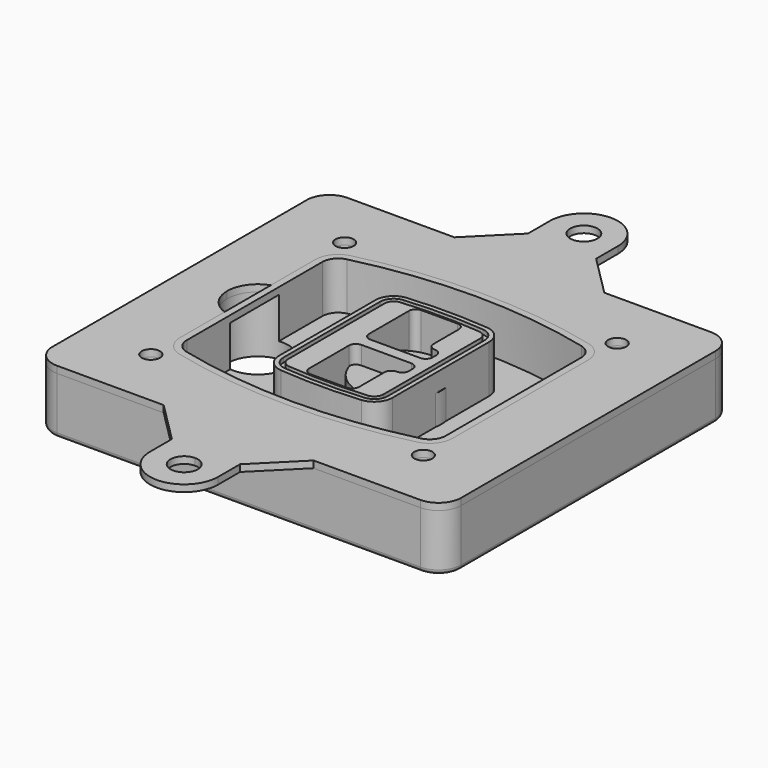
from build123d import *

# Parameters (mm, degrees)
F0_R      = 4
F1_DEPTH  = 25
F2_DEPTH  = 3
F3_DEPTH  = 18
F5_DEPTH  = 21
F6_DEPTH  = 2
F8_DEPTH  = 20
F9_DEPTH  = 16
F10_DEPTH = 25
F7_R      = 6
F7_R_2    = 4
F11_DEPTH = 6
F13_DEPTH = 9
F15_R     = 2
F17_DEPTH = 3
F16_R     = 4
F18_DEPTH = 3


# Not quite as in the source:
# - a feature of the source that left no trace in its solid (it failed there, or was rolled back) is left out
# - a feature names something its author has since deleted; it is built from what else it names


with BuildPart() as f1:
    # F0 (on Top) → F1 (new body)
    with BuildSketch(Plane.XY):
        with BuildLine():
            ThreePointArc((-90, -70), (-87.0710678119, -77.0710678119), (-80, -80))
            Line((-80, -80), (80, -80))
            ThreePointArc((80, -80), (87.0710678119, -77.0710678119), (90, -70))
            Line((90, -70), (90, 70))
            ThreePointArc((90, 70), (87.0710678119, 77.0710678119), (80, 80))
            Line((80, 80), (-80, 80))
            ThreePointArc((-80, 80), (-87.0710678119, 77.0710678119), (-90, 70))
            Line((-90, 70), (-90, -70))
        make_face()
        with Locations((-60, -53.3333333333)):
            Circle(F0_R, mode=Mode.SUBTRACT)
        with Locations((60, -53.3333333333)):
            Circle(F0_R, mode=Mode.SUBTRACT)
        with Locations((-60, 53.3333333333)):
            Circle(F0_R, mode=Mode.SUBTRACT)
        with BuildLine():
            ThreePointArc((-64, 37.2990447398), (-61.0143011354, 45.9411029726), (-53.3306899286, 50.8970778549))
            ThreePointArc((-53.3306899286, 50.8970778549), (0, 57.3333333333), (53.3306899286, 50.8970778549))
            ThreePointArc((53.3306899286, 50.8970778549), (61.0143011354, 45.9411029726), (64, 37.2990447398))
            Line((64, 37.2990447398), (64, -37.2990447398))
            ThreePointArc((64, -37.2990447398), (61.0143011354, -45.9411029726), (53.3306899286, -50.8970778549))
            ThreePointArc((53.3306899286, -50.8970778549), (0, -57.3333333333), (-53.3306899286, -50.8970778549))
            ThreePointArc((-53.3306899286, -50.8970778549), (-61.0143011354, -45.9411029726), (-64, -37.2990447398))
            Line((-64, -37.2990447398), (-64, 37.2990447398))
        make_face(mode=Mode.SUBTRACT)
        with Locations((60, 53.3333333333)):
            Circle(F0_R, mode=Mode.SUBTRACT)
        with BuildLine():
            ThreePointArc((53.3306899286, 50.8970778549), (0, 57.3333333333), (-53.3306899286, 50.8970778549))
            ThreePointArc((-53.3306899286, 50.8970778549), (-61.0143011354, 45.9411029726), (-64, 37.2990447398))
            Line((-64, 37.2990447398), (-64, -37.2990447398))
            ThreePointArc((-64, -37.2990447398), (-61.0143011354, -45.9411029726), (-53.3306899286, -50.8970778549))
            ThreePointArc((-53.3306899286, -50.8970778549), (0, -57.3333333333), (53.3306899286, -50.8970778549))
            ThreePointArc((53.3306899286, -50.8970778549), (61.0143011354, -45.9411029726), (64, -37.2990447398))
            Line((64, -37.2990447398), (64, 37.2990447398))
            ThreePointArc((64, 37.2990447398), (61.0143011354, 45.9411029726), (53.3306899286, 50.8970778549))
        make_face()
        with BuildLine():
            Line((-60, -37.2990447398), (-60, 37.2990447398))
            ThreePointArc((-60, 37.2990447398), (-57.8673579538, 43.4719434775), (-52.3790642347, 47.0119255363))
            ThreePointArc((-52.3790642347, 47.0119255363), (0, 53.3333333333), (52.3790642347, 47.0119255363))
            ThreePointArc((52.3790642347, 47.0119255363), (57.8673579538, 43.4719434775), (60, 37.2990447398))
            Line((60, 37.2990447398), (60, -37.2990447398))
            ThreePointArc((60, -37.2990447398), (57.8673579538, -43.4719434775), (52.3790642347, -47.0119255363))
            ThreePointArc((52.3790642347, -47.0119255363), (0, -53.3333333333), (-52.3790642347, -47.0119255363))
            ThreePointArc((-52.3790642347, -47.0119255363), (-57.8673579538, -43.4719434775), (-60, -37.2990447398))
        make_face(mode=Mode.SUBTRACT)
        with BuildLine():
            ThreePointArc((-52.3790642347, 47.0119255363), (-57.8673579538, 43.4719434775), (-60, 37.2990447398))
            Line((-60, 37.2990447398), (-60, -37.2990447398))
            ThreePointArc((-60, -37.2990447398), (-57.8673579538, -43.4719434775), (-52.3790642347, -47.0119255363))
            ThreePointArc((-52.3790642347, -47.0119255363), (0, -53.3333333333), (52.3790642347, -47.0119255363))
            ThreePointArc((52.3790642347, -47.0119255363), (57.8673579538, -43.4719434775), (60, -37.2990447398))
            Line((60, -37.2990447398), (60, 37.2990447398))
            ThreePointArc((60, 37.2990447398), (57.8673579538, 43.4719434775), (52.3790642347, 47.0119255363))
            ThreePointArc((52.3790642347, 47.0119255363), (0, 53.3333333333), (-52.3790642347, 47.0119255363))
        make_face()
        with BuildLine():
            ThreePointArc((51.6653449643, 44.0980612973), (55.5071505677, 41.6200738562), (57, 37.2990447398))
            Line((57, 37.2990447398), (57, -37.2990447398))
            ThreePointArc((57, -37.2990447398), (55.5071505677, -41.6200738562), (51.6653449643, -44.0980612973))
            ThreePointArc((51.6653449643, -44.0980612973), (0, -50.3333333333), (-51.6653449643, -44.0980612973))
            ThreePointArc((-51.6653449643, -44.0980612973), (-55.5071505677, -41.6200738562), (-57, -37.2990447398))
            Line((-57, -37.2990447398), (-57, 37.2990447398))
            ThreePointArc((-57, 37.2990447398), (-55.5071505677, 41.6200738562), (-51.6653449643, 44.0980612973))
            ThreePointArc((-51.6653449643, 44.0980612973), (0, 50.3333333333), (51.6653449643, 44.0980612973))
        make_face(mode=Mode.SUBTRACT)
        with BuildLine():
            Line((57, -37.2990447398), (57, 37.2990447398))
            ThreePointArc((57, 37.2990447398), (55.5071505677, 41.6200738562), (51.6653449643, 44.0980612973))
            ThreePointArc((51.6653449643, 44.0980612973), (0, 50.3333333333), (-51.6653449643, 44.0980612973))
            ThreePointArc((-51.6653449643, 44.0980612973), (-55.5071505677, 41.6200738562), (-57, 37.2990447398))
            Line((-57, 37.2990447398), (-57, -37.2990447398))
            ThreePointArc((-57, -37.2990447398), (-55.5071505677, -41.6200738562), (-51.6653449643, -44.0980612973))
            ThreePointArc((-51.6653449643, -44.0980612973), (0, -50.3333333333), (51.6653449643, -44.0980612973))
            ThreePointArc((51.6653449643, -44.0980612973), (55.5071505677, -41.6200738562), (57, -37.2990447398))
        make_face()
    extrude(amount=-F1_DEPTH)

    # F0 (on Top) → F2 (join)
    with BuildSketch(Plane.XY):
        with BuildLine():
            ThreePointArc((-52.3790642347, 47.0119255363), (-57.8673579538, 43.4719434775), (-60, 37.2990447398))
            Line((-60, 37.2990447398), (-60, -37.2990447398))
            ThreePointArc((-60, -37.2990447398), (-57.8673579538, -43.4719434775), (-52.3790642347, -47.0119255363))
            ThreePointArc((-52.3790642347, -47.0119255363), (0, -53.3333333333), (52.3790642347, -47.0119255363))
            ThreePointArc((52.3790642347, -47.0119255363), (57.8673579538, -43.4719434775), (60, -37.2990447398))
            Line((60, -37.2990447398), (60, 37.2990447398))
            ThreePointArc((60, 37.2990447398), (57.8673579538, 43.4719434775), (52.3790642347, 47.0119255363))
            ThreePointArc((52.3790642347, 47.0119255363), (0, 53.3333333333), (-52.3790642347, 47.0119255363))
        make_face()
        with BuildLine():
            ThreePointArc((51.6653449643, 44.0980612973), (55.5071505677, 41.6200738562), (57, 37.2990447398))
            Line((57, 37.2990447398), (57, -37.2990447398))
            ThreePointArc((57, -37.2990447398), (55.5071505677, -41.6200738562), (51.6653449643, -44.0980612973))
            ThreePointArc((51.6653449643, -44.0980612973), (0, -50.3333333333), (-51.6653449643, -44.0980612973))
            ThreePointArc((-51.6653449643, -44.0980612973), (-55.5071505677, -41.6200738562), (-57, -37.2990447398))
            Line((-57, -37.2990447398), (-57, 37.2990447398))
            ThreePointArc((-57, 37.2990447398), (-55.5071505677, 41.6200738562), (-51.6653449643, 44.0980612973))
            ThreePointArc((-51.6653449643, 44.0980612973), (0, 50.3333333333), (51.6653449643, 44.0980612973))
        make_face(mode=Mode.SUBTRACT)
    extrude(amount=F2_DEPTH)

    # F0 (on Top) → F3 (cut)
    with BuildSketch(Plane.XY):
        with BuildLine():
            Line((57, -37.2990447398), (57, 37.2990447398))
            ThreePointArc((57, 37.2990447398), (55.5071505677, 41.6200738562), (51.6653449643, 44.0980612973))
            ThreePointArc((51.6653449643, 44.0980612973), (0, 50.3333333333), (-51.6653449643, 44.0980612973))
            ThreePointArc((-51.6653449643, 44.0980612973), (-55.5071505677, 41.6200738562), (-57, 37.2990447398))
            Line((-57, 37.2990447398), (-57, -37.2990447398))
            ThreePointArc((-57, -37.2990447398), (-55.5071505677, -41.6200738562), (-51.6653449643, -44.0980612973))
            ThreePointArc((-51.6653449643, -44.0980612973), (0, -50.3333333333), (51.6653449643, -44.0980612973))
            ThreePointArc((51.6653449643, -44.0980612973), (55.5071505677, -41.6200738562), (57, -37.2990447398))
        make_face()
    extrude(amount=-F3_DEPTH, mode=Mode.SUBTRACT)

    # F4 (on face) → F5 (join, through all)
    with BuildSketch(Plane.XY.offset(3)):
        with BuildLine():
            ThreePointArc((-25, -26.587695628), (-22.8992979869, -31.9912392117), (-17.7004291845, -34.5569740744))
            ThreePointArc((-17.7004291845, -34.5569740744), (0, -35.3333333333), (17.7004291845, -34.5569740744))
            ThreePointArc((17.7004291845, -34.5569740744), (22.8992979869, -31.9912392117), (25, -26.587695628))
            Line((25, -26.587695628), (25, 26.587695628))
            ThreePointArc((25, 26.587695628), (22.8992979869, 31.9912392117), (17.7004291845, 34.5569740744))
            ThreePointArc((17.7004291845, 34.5569740744), (0, 35.3333333333), (-17.7004291845, 34.5569740744))
            ThreePointArc((-17.7004291845, 34.5569740744), (-22.8992979869, 31.9912392117), (-25, 26.587695628))
            Line((-25, 26.587695628), (-25, -26.587695628))
        make_face()
        with BuildLine():
            ThreePointArc((17.5253218884, 32.5646544628), (21.4244734902, 30.6403533158), (23, 26.587695628))
            Line((23, 26.587695628), (23, -26.587695628))
            ThreePointArc((23, -26.587695628), (21.4244734902, -30.6403533158), (17.5253218884, -32.5646544628))
            ThreePointArc((17.5253218884, -32.5646544628), (0, -33.3333333333), (-17.5253218884, -32.5646544628))
            ThreePointArc((-17.5253218884, -32.5646544628), (-21.4244734902, -30.6403533158), (-23, -26.587695628))
            Line((-23, -26.587695628), (-23, 26.587695628))
            ThreePointArc((-23, 26.587695628), (-21.4244734902, 30.6403533158), (-17.5253218884, 32.5646544628))
            ThreePointArc((-17.5253218884, 32.5646544628), (0, 33.3333333333), (17.5253218884, 32.5646544628))
        make_face(mode=Mode.SUBTRACT)
        with BuildLine():
            Line((23, -26.587695628), (23, 26.587695628))
            ThreePointArc((23, 26.587695628), (21.4244734902, 30.6403533158), (17.5253218884, 32.5646544628))
            ThreePointArc((17.5253218884, 32.5646544628), (0, 33.3333333333), (-17.5253218884, 32.5646544628))
            ThreePointArc((-17.5253218884, 32.5646544628), (-21.4244734902, 30.6403533158), (-23, 26.587695628))
            Line((-23, 26.587695628), (-23, -26.587695628))
            ThreePointArc((-23, -26.587695628), (-21.4244734902, -30.6403533158), (-17.5253218884, -32.5646544628))
            ThreePointArc((-17.5253218884, -32.5646544628), (0, -33.3333333333), (17.5253218884, -32.5646544628))
            ThreePointArc((17.5253218884, -32.5646544628), (21.4244734902, -30.6403533158), (23, -26.587695628))
        make_face()
        with BuildLine():
            ThreePointArc((17.3502145923, 30.5723348512), (19.9496489934, 29.2894674198), (21, 26.587695628))
            Line((21, 26.587695628), (21, -26.587695628))
            ThreePointArc((21, -26.587695628), (19.9496489934, -29.2894674198), (17.3502145923, -30.5723348512))
            ThreePointArc((17.3502145923, -30.5723348512), (0, -31.3333333333), (-17.3502145923, -30.5723348512))
            ThreePointArc((-17.3502145923, -30.5723348512), (-19.9496489934, -29.2894674198), (-21, -26.587695628))
            Line((-21, -26.587695628), (-21, 26.587695628))
            ThreePointArc((-21, 26.587695628), (-19.9496489934, 29.2894674198), (-17.3502145923, 30.5723348512))
            ThreePointArc((-17.3502145923, 30.5723348512), (0, 31.3333333333), (17.3502145923, 30.5723348512))
        make_face(mode=Mode.SUBTRACT)
        with BuildLine():
            Line((21, -26.587695628), (21, 26.587695628))
            ThreePointArc((21, 26.587695628), (19.9496489934, 29.2894674198), (17.3502145923, 30.5723348512))
            ThreePointArc((17.3502145923, 30.5723348512), (0, 31.3333333333), (-17.3502145923, 30.5723348512))
            ThreePointArc((-17.3502145923, 30.5723348512), (-19.9496489934, 29.2894674198), (-21, 26.587695628))
            Line((-21, 26.587695628), (-21, -26.587695628))
            ThreePointArc((-21, -26.587695628), (-19.9496489934, -29.2894674198), (-17.3502145923, -30.5723348512))
            ThreePointArc((-17.3502145923, -30.5723348512), (0, -31.3333333333), (17.3502145923, -30.5723348512))
            ThreePointArc((17.3502145923, -30.5723348512), (19.9496489934, -29.2894674198), (21, -26.587695628))
        make_face()
        with BuildLine():
            Line((-8, -2.5), (14, -2.5))
            ThreePointArc((14, -2.5), (16.1213203436, -3.3786796564), (17, -5.5))
            Line((17, -5.5), (17, -7.5))
            ThreePointArc((17, -7.5), (16.1213203436, -9.6213203436), (14, -10.5))
            ThreePointArc((14, -10.5), (11.8786796564, -11.3786796564), (11, -13.5))
            Line((11, -13.5), (11, -27.5))
            ThreePointArc((11, -27.5), (10.1213203436, -29.6213203436), (8, -30.5))
            Line((8, -30.5), (-8, -30.5))
            ThreePointArc((-8, -30.5), (-10.1213203436, -29.6213203436), (-11, -27.5))
            Line((-11, -27.5), (-11, -5.5))
            ThreePointArc((-11, -5.5), (-10.1213203436, -3.3786796564), (-8, -2.5))
        make_face(mode=Mode.SUBTRACT)
        with BuildLine():
            ThreePointArc((-8, 2.5), (-10.1213203436, 3.3786796564), (-11, 5.5))
            Line((-11, 5.5), (-11, 27.5))
            ThreePointArc((-11, 27.5), (-10.1213203436, 29.6213203436), (-8, 30.5))
            Line((-8, 30.5), (8, 30.5))
            ThreePointArc((8, 30.5), (10.1213203436, 29.6213203436), (11, 27.5))
            Line((11, 27.5), (11, 13.5))
            ThreePointArc((11, 13.5), (11.8786796564, 11.3786796564), (14, 10.5))
            ThreePointArc((14, 10.5), (16.1213203436, 9.6213203436), (17, 7.5))
            Line((17, 7.5), (17, 5.5))
            ThreePointArc((17, 5.5), (16.1213203436, 3.3786796564), (14, 2.5))
            Line((14, 2.5), (-8, 2.5))
        make_face(mode=Mode.SUBTRACT)
    extrude(amount=-F5_DEPTH)

    # F4 (on face) → F6 (cut)
    with BuildSketch(Plane.XY.offset(3)):
        with BuildLine():
            Line((23, -26.587695628), (23, 26.587695628))
            ThreePointArc((23, 26.587695628), (21.4244734902, 30.6403533158), (17.5253218884, 32.5646544628))
            ThreePointArc((17.5253218884, 32.5646544628), (0, 33.3333333333), (-17.5253218884, 32.5646544628))
            ThreePointArc((-17.5253218884, 32.5646544628), (-21.4244734902, 30.6403533158), (-23, 26.587695628))
            Line((-23, 26.587695628), (-23, -26.587695628))
            ThreePointArc((-23, -26.587695628), (-21.4244734902, -30.6403533158), (-17.5253218884, -32.5646544628))
            ThreePointArc((-17.5253218884, -32.5646544628), (0, -33.3333333333), (17.5253218884, -32.5646544628))
            ThreePointArc((17.5253218884, -32.5646544628), (21.4244734902, -30.6403533158), (23, -26.587695628))
        make_face()
        with BuildLine():
            ThreePointArc((17.3502145923, 30.5723348512), (19.9496489934, 29.2894674198), (21, 26.587695628))
            Line((21, 26.587695628), (21, -26.587695628))
            ThreePointArc((21, -26.587695628), (19.9496489934, -29.2894674198), (17.3502145923, -30.5723348512))
            ThreePointArc((17.3502145923, -30.5723348512), (0, -31.3333333333), (-17.3502145923, -30.5723348512))
            ThreePointArc((-17.3502145923, -30.5723348512), (-19.9496489934, -29.2894674198), (-21, -26.587695628))
            Line((-21, -26.587695628), (-21, 26.587695628))
            ThreePointArc((-21, 26.587695628), (-19.9496489934, 29.2894674198), (-17.3502145923, 30.5723348512))
            ThreePointArc((-17.3502145923, 30.5723348512), (0, 31.3333333333), (17.3502145923, 30.5723348512))
        make_face(mode=Mode.SUBTRACT)
    extrude(amount=-F6_DEPTH, mode=Mode.SUBTRACT)

    # F7 (on face) → F8 (join)
    with BuildSketch(Plane(origin=(0, 0, -25), x_dir=(1, 0, 0), z_dir=(0, 0, -1))):
        with BuildLine():
            ThreePointArc((-6.71157564, 0), (6.7567035675, 13.4682792075), (20.224982775, 0))
            Line((20.224982775, 0), (25.224982775, 0))
            ThreePointArc((25.224982775, 0), (6.7567035675, 18.4682792075), (-11.71157564, 0))
            Line((-11.71157564, 0), (-6.71157564, 0))
        make_face()
        with BuildLine():
            Line((-6.71157564, 0), (20.224982775, 0))
            ThreePointArc((20.224982775, 0), (6.7567035675, 13.4682792075), (-6.71157564, 0))
        make_face()
        with BuildLine():
            ThreePointArc((-6.71157564, 0), (6.7567035675, -13.4682792075), (20.224982775, 0))
            Line((20.224982775, 0), (-6.71157564, 0))
        make_face()
        with BuildLine():
            Line((25.224982775, 0), (20.224982775, 0))
            ThreePointArc((20.224982775, 0), (6.7567035675, -13.4682792075), (-6.71157564, 0))
            Line((-6.71157564, 0), (-11.71157564, 0))
            ThreePointArc((-11.71157564, 0), (6.7567035675, -18.4682792075), (25.224982775, 0))
        make_face()
    extrude(amount=-F8_DEPTH)

    # F7 (on face) → F9 (cut)
    with BuildSketch(Plane(origin=(0, 0, -25), x_dir=(1, 0, 0), z_dir=(0, 0, -1))):
        with BuildLine():
            Line((-6.71157564, 0), (20.224982775, 0))
            ThreePointArc((20.224982775, 0), (6.7567035675, 13.4682792075), (-6.71157564, 0))
        make_face()
        with BuildLine():
            ThreePointArc((-6.71157564, 0), (6.7567035675, -13.4682792075), (20.224982775, 0))
            Line((20.224982775, 0), (-6.71157564, 0))
        make_face()
    extrude(amount=-F9_DEPTH, mode=Mode.SUBTRACT)

    # F7 (on face) → F10 (cut)
    with BuildSketch(Plane(origin=(0, 0, -25), x_dir=(1, 0, 0), z_dir=(0, 0, -1))):
        with BuildLine():
            Line((-69.0318229325, 0), (-42.0952645175, 0))
            ThreePointArc((-42.0952645175, 0), (-55.563543725, 13.4682792075), (-69.0318229325, 0))
        make_face()
        with BuildLine():
            ThreePointArc((-69.0318229325, 0), (-55.563543725, -13.4682792075), (-42.0952645175, 0))
            Line((-42.0952645175, 0), (-69.0318229325, 0))
        make_face()
    extrude(amount=-F10_DEPTH, mode=Mode.SUBTRACT)

    # F7 (on face) → F11 (cut)
    with BuildSketch(Plane(origin=(0, 0, -25), x_dir=(1, 0, 0), z_dir=(0, 0, -1))):
        with Locations((60, -53.3333333333)):
            Circle(F7_R)
        with Locations((60, -53.3333333333)):
            Circle(F7_R_2, mode=Mode.SUBTRACT)
        with Locations((-60, -53.3333333333)):
            Circle(F7_R)
        with Locations((-60, -53.3333333333)):
            Circle(F7_R_2, mode=Mode.SUBTRACT)
        with Locations((-60, 53.3333333333)):
            Circle(F7_R)
        with Locations((-60, 53.3333333333)):
            Circle(F7_R_2, mode=Mode.SUBTRACT)
        with Locations((60, 53.3333333333)):
            Circle(F7_R)
        with Locations((60, 53.3333333333)):
            Circle(F7_R_2, mode=Mode.SUBTRACT)
    extrude(amount=-F11_DEPTH, mode=Mode.SUBTRACT)

    # F12 (on face) → F13 (cut, through all)
    with BuildSketch(Plane(origin=(0, 0, -9), x_dir=(1, 0, 0), z_dir=(0, 0, -1))):
        with BuildLine():
            ThreePointArc((20.224982775, 0), (20.1663399806, 1.2554664788), (19.9909222755, 2.5))
            Line((19.9909222755, 2.5), (14, 2.5))
            ThreePointArc((14, 2.5), (16.1213203436, 3.3786796564), (17, 5.5))
            Line((17, 5.5), (17, 7.5))
            ThreePointArc((17, 7.5), (16.1213203436, 9.6213203436), (14, 10.5))
            ThreePointArc((14, 10.5), (12.1627255951, 11.1284134507), (11.0951631559, 12.750384826))
            ThreePointArc((11.0951631559, 12.750384826), (11.0476113807, 12.7664660322), (11, 12.7823698976))
            Line((11, 12.7823698976), (11, -12.7823698976))
            ThreePointArc((11, -12.7823698976), (11.0476113807, -12.7664660322), (11.0951631559, -12.750384826))
            ThreePointArc((11.0951631559, -12.750384826), (12.1627255951, -11.1284134507), (14, -10.5))
            ThreePointArc((14, -10.5), (16.1213203436, -9.6213203436), (17, -7.5))
            Line((17, -7.5), (17, -5.5))
            ThreePointArc((17, -5.5), (16.1213203436, -3.3786796564), (14, -2.5))
            Line((14, -2.5), (19.9909222755, -2.5))
            ThreePointArc((19.9909222755, -2.5), (20.1663399806, -1.2554664788), (20.224982775, 0))
        make_face()
    extrude(amount=F13_DEPTH, mode=Mode.SUBTRACT)

    # F15
    f15_edges = [f1.edges().sort_by_distance(p)[0] for p in [
        (0, -80, -25),
        (-87.071068, -77.071068, -25),
        (-90, 0, -25),
        (-87.071068, 77.071068, -25),
        (87.071068, -77.071068, -25),
        (0, 80, -25),
        (90, 0, -25),
        (87.071068, 77.071068, -25),
    ]]
    fillet(f15_edges, radius=F15_R)


with BuildPart() as f17:
    # F16 (on face) → F17 (new body, through all)
    with BuildSketch(Plane.XY):
        with BuildLine():
            Line((-15, 98), (-33, 80))
            Line((-33, 80), (0, 80))
            Line((0, 80), (33, 80))
            Line((33, 80), (15, 98))
            Line((15, 98), (15, 110))
            ThreePointArc((15, 110), (0, 125), (-15, 110))
            Line((-15, 110), (-15, 98))
        make_face()
        with BuildLine():
            ThreePointArc((6, 110), (4.2426406871, 105.7573593129), (0, 104))
            ThreePointArc((0, 104), (-4.2426406871, 114.2426406871), (6, 110))
        make_face(mode=Mode.SUBTRACT)
    extrude(amount=F17_DEPTH)



with BuildPart() as f17b:
    # F16 (on face) → F17, piece 2 (new body, through all)
    with BuildSketch(Plane.XY):
        with BuildLine():
            Line((0, -80), (-33, -80))
            Line((-33, -80), (-15, -98))
            Line((-15, -98), (-15, -110))
            ThreePointArc((-15, -110), (0, -125), (15, -110))
            Line((15, -110), (15, -98))
            Line((15, -98), (33, -80))
            Line((33, -80), (0, -80))
        make_face()
        with BuildLine():
            ThreePointArc((6, -110), (-4.2426406871, -114.2426406871), (0, -104))
            ThreePointArc((0, -104), (4.2426406871, -105.7573593129), (6, -110))
        make_face(mode=Mode.SUBTRACT)
    extrude(amount=F17_DEPTH)


with BuildPart() as f17_1:
    add(f17.part)

    add(f17b.part)  # F18 merges F17b
    # F16 (on face) → F18 (join, through all)
    with BuildSketch(Plane.XY):
        with BuildLine():
            Line((-33, 80), (-80, 80))
            ThreePointArc((-80, 80), (-87.0710678119, 77.0710678119), (-90, 70))
            Line((-90, 70), (-90, -70))
            ThreePointArc((-90, -70), (-87.0710678119, -77.0710678119), (-80, -80))
            Line((-80, -80), (-33, -80))
            Line((-33, -80), (0, -80))
            Line((0, -80), (33, -80))
            Line((33, -80), (80, -80))
            ThreePointArc((80, -80), (87.0710678119, -77.0710678119), (90, -70))
            Line((90, -70), (90, 70))
            ThreePointArc((90, 70), (87.0710678119, 77.0710678119), (80, 80))
            Line((80, 80), (33, 80))
            Line((33, 80), (0, 80))
            Line((0, 80), (-33, 80))
        make_face()
        with Locations((-60, -53.3333333333)):
            Circle(F16_R, mode=Mode.SUBTRACT)
        with Locations((60, -53.3333333333)):
            Circle(F16_R, mode=Mode.SUBTRACT)
        with Locations((-60, 53.3333333333)):
            Circle(F16_R, mode=Mode.SUBTRACT)
        with BuildLine():
            ThreePointArc((-52.3790642347, 47.0119255363), (0, 53.3333333333), (52.3790642347, 47.0119255363))
            ThreePointArc((52.3790642347, 47.0119255363), (57.8673579538, 43.4719434775), (60, 37.2990447398))
            Line((60, 37.2990447398), (60, -37.2990447398))
            ThreePointArc((60, -37.2990447398), (57.8673579538, -43.4719434775), (52.3790642347, -47.0119255363))
            ThreePointArc((52.3790642347, -47.0119255363), (0, -53.3333333333), (-52.3790642347, -47.0119255363))
            ThreePointArc((-52.3790642347, -47.0119255363), (-57.8673579538, -43.4719434775), (-60, -37.2990447398))
            Line((-60, -37.2990447398), (-60, -12.7166190685))
            ThreePointArc((-60, -12.7166190685), (-66.5441169481, -7.798817635), (-69.0318229325, 0))
            ThreePointArc((-69.0318229325, 0), (-66.5441169481, 7.798817635), (-60, 12.7166190685))
            Line((-60, 12.7166190685), (-60, 37.2990447398))
            ThreePointArc((-60, 37.2990447398), (-57.8673579538, 43.4719434775), (-52.3790642347, 47.0119255363))
        make_face(mode=Mode.SUBTRACT)
        with Locations((60, 53.3333333333)):
            Circle(F16_R, mode=Mode.SUBTRACT)
    extrude(amount=F18_DEPTH)


solid = Compound([f1.part, f17_1.part])
